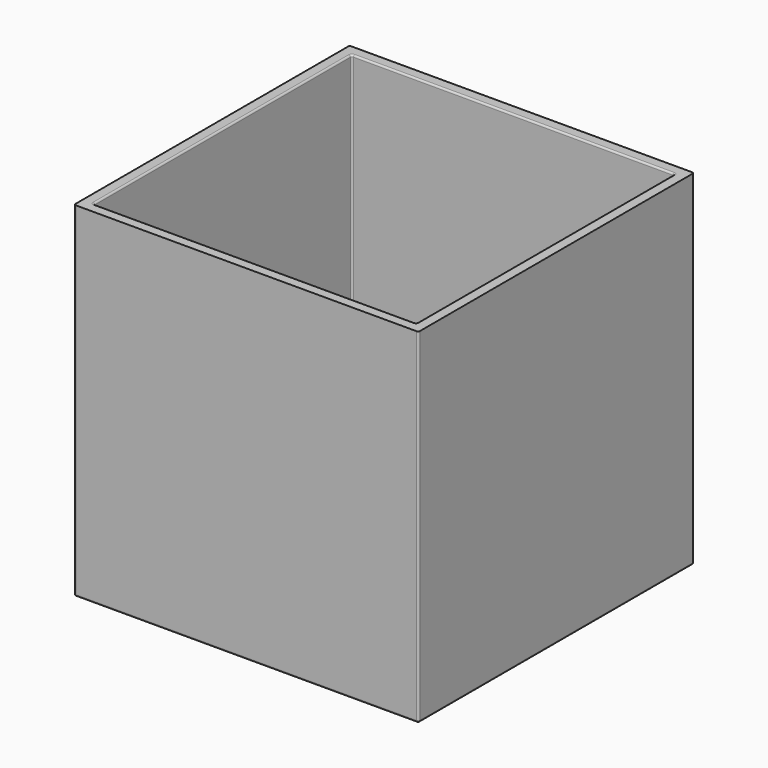
from build123d import *

# Parameters (mm, degrees)
F0_W         = 50.8
F0_H         = 50.8
F1_DEPTH     = 1.5875
F2_W         = 50.8
F2_H         = 50.8
F2_W_2       = 47.625
F2_H_2       = 47.625
F3_DEPTH     = 49.2125
F4_R         = 0.254
F5_TEXT_SIZE = 10.6758734567
F6_DEPTH     = 0.254


# Not quite as in the source:
# - Text() gives the source's letters only with a copy of the font that has no kerning and outlines rounded to 1/6400 em; it was checked with that copy


with BuildPart() as f1:
    # F0 (on Top) → F1 (new body)
    with BuildSketch(Plane.XY):
        Rectangle(F0_W, F0_H)
    extrude(amount=F1_DEPTH)

    # F2 (on face) → F3 (join)
    with BuildSketch(Plane.XY.offset(1.5875)):
        Rectangle(F2_W, F2_H)
        Rectangle(F2_W_2, F2_H_2, mode=Mode.SUBTRACT)
    extrude(amount=F3_DEPTH)

    # F4
    f4_edges = [f1.edges().sort_by_distance(p)[0] for p in [
        (-23.8125, 0, 1.5875),
        (-23.8125, -23.8125, 26.19375),
        (0, -23.8125, 1.5875),
        (-23.8125, 0, 50.8),
        (0, -23.8125, 50.8),
        (0, 23.8125, 1.5875),
        (-23.8125, 23.8125, 26.19375),
        (0, 23.8125, 50.8),
        (23.8125, 23.8125, 26.19375),
        (23.8125, 0, 1.5875),
        (23.8125, 0, 50.8),
        (23.8125, -23.8125, 26.19375),
        (-25.4, -25.4, 25.4),
        (25.4, -25.4, 25.4),
        (25.4, 25.4, 25.4),
        (-25.4, 25.4, 25.4),
        (-25.4, 0, 0),
        (0, -25.4, 0),
        (0, 25.4, 0),
        (25.4, 0, 0),
    ]]
    fillet(f4_edges, radius=F4_R)

    # F5 (on face) → F6 (cut)
    with BuildSketch(Plane(origin=(0, 25.4, 0), x_dir=(-1, 0, 0), z_dir=(0, 1, 0))):
        with Locations((-22.225, 30.4133711112)):
            Text('Breakers', F5_TEXT_SIZE, font='Open Sans', text_align=(TextAlign.LEFT, TextAlign.BOTTOM))
    extrude(amount=-F6_DEPTH, mode=Mode.SUBTRACT)


solid = f1.part
